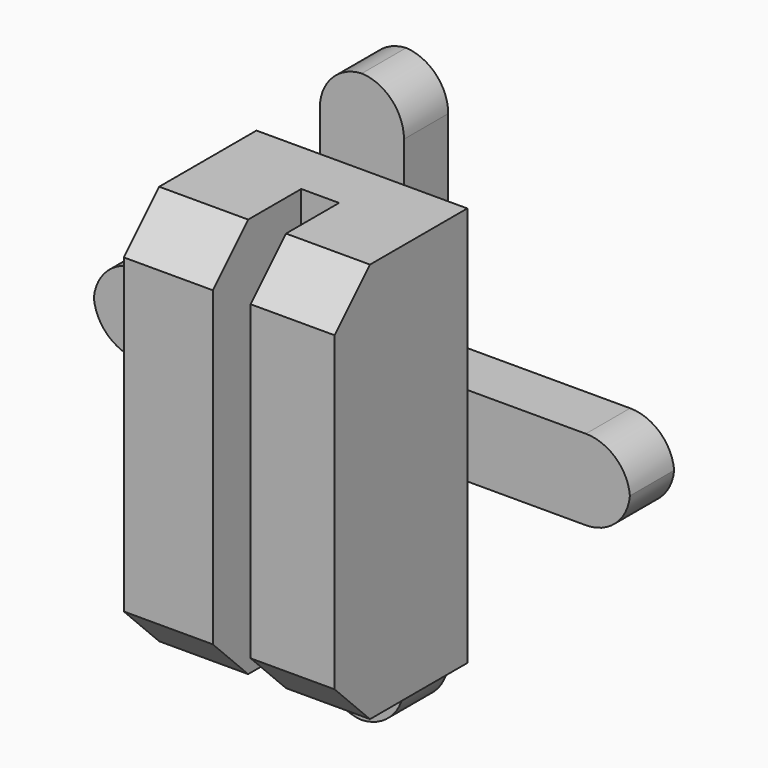
from build123d import *

# Parameters (mm, degrees)
F0_W        = 19.3394050002
F0_H        = 56.1432316899
F0_W_2      = 51.9402250648
F0_H_2      = 18.5019075871
F1_DEPTH    = 12.7
F2_T1_DEPTH = 63.5
F3_W        = 48.4298244119
F3_H        = 91.9232070446
F4_DEPTH    = 12.7
F5_W        = 20.4465882853
F5_H        = 91.9232070446
F5_W_2      = 19.2932416685
F6_DEPTH    = 25.4
F7_SIZE     = 10.16


# Not quite as in the source:
# - a fillet or chamfer that OpenCascade refuses, or shapes differently, is made with other operations: its cross-section is extruded or revolved along the edge and cut away or added


with BuildPart() as f1:
    # F0 (on Front) → F1 (new body)
    with BuildSketch(Plane.XZ):
        with Locations((0, 37.3225696385)):
            Rectangle(F0_W, F0_H)
        with Locations((35.6398150325, 0)):
            Rectangle(F0_W_2, F0_H_2)
        Rectangle(F0_W, F0_H_2)
        with Locations((-35.6398150325, 0)):
            Rectangle(F0_W_2, F0_H_2)
        with Locations((0, -37.3225696385)):
            Rectangle(F0_W, F0_H)
    extrude(amount=F1_DEPTH)

    # F2: fillet of radius 10.16 on 8 edges, made by hand

    # F2_s2 → F2_t1 (cut)
    with BuildSketch(Plane.XZ.offset(-25.4)):
        with BuildLine():
            ThreePointArc((9.6697025001, 55.2341854835), (6.693907397, 62.4183903803), (-0.4902974999, 65.3941854835))
            Line((-0.4902974999, 65.3941854835), (9.6697025001, 65.3941854835))
            Line((9.6697025001, 65.3941854835), (9.6697025001, 55.2341854835))
        make_face()
        with BuildLine():
            ThreePointArc((0.4902974999, 65.3941854835), (-6.693907397, 62.4183903803), (-9.6697025001, 55.2341854835))
            Line((-9.6697025001, 55.2341854835), (-9.6697025001, 65.3941854835))
            Line((-9.6697025001, 65.3941854835), (0.4902974999, 65.3941854835))
        make_face()
        with BuildLine():
            ThreePointArc((61.6099275649, -0.9090462065), (58.6341324617, 6.2751586904), (51.4499275649, 9.2509537935))
            Line((51.4499275649, 9.2509537935), (61.6099275649, 9.2509537935))
            Line((61.6099275649, 9.2509537935), (61.6099275649, -0.9090462065))
        make_face()
        with BuildLine():
            ThreePointArc((51.4499275649, -9.2509537935), (58.6341324617, -6.2751586904), (61.6099275649, 0.9090462065))
            Line((61.6099275649, 0.9090462065), (61.6099275649, -9.2509537935))
            Line((61.6099275649, -9.2509537935), (51.4499275649, -9.2509537935))
        make_face()
        with BuildLine():
            ThreePointArc((-0.4902974999, -65.3941854835), (6.693907397, -62.4183903803), (9.6697025001, -55.2341854835))
            Line((9.6697025001, -55.2341854835), (9.6697025001, -65.3941854835))
            Line((9.6697025001, -65.3941854835), (-0.4902974999, -65.3941854835))
        make_face()
        with BuildLine():
            ThreePointArc((-51.4499275649, 9.2509537935), (-58.6341324617, 6.2751586904), (-61.6099275649, -0.9090462065))
            Line((-61.6099275649, -0.9090462065), (-61.6099275649, 9.2509537935))
            Line((-61.6099275649, 9.2509537935), (-51.4499275649, 9.2509537935))
        make_face()
        with BuildLine():
            ThreePointArc((-61.6099275649, 0.9090462065), (-58.6341324617, -6.2751586904), (-51.4499275649, -9.2509537935))
            Line((-51.4499275649, -9.2509537935), (-61.6099275649, -9.2509537935))
            Line((-61.6099275649, -9.2509537935), (-61.6099275649, 0.9090462065))
        make_face()
        with BuildLine():
            ThreePointArc((-9.6697025001, -55.2341854835), (-6.693907397, -62.4183903803), (0.4902974999, -65.3941854835))
            Line((0.4902974999, -65.3941854835), (-9.6697025001, -65.3941854835))
            Line((-9.6697025001, -65.3941854835), (-9.6697025001, -55.2341854835))
        make_face()
    extrude(amount=F2_T1_DEPTH, mode=Mode.SUBTRACT)

    # F3 (on face) → F4 (join)
    with BuildSketch(Plane.XZ.offset(12.7)):
        Rectangle(F3_W, F3_H)
    extrude(amount=F4_DEPTH)

    # F5 (on face) → F6 (join)
    with BuildSketch(Plane.XZ.offset(25.4)):
        with Locations((-13.9916180633, 0)):
            Rectangle(F5_W, F5_H)
        with Locations((14.5682913717, 0)):
            Rectangle(F5_W_2, F5_H)
    extrude(amount=F6_DEPTH)

    # F7
    f7_edges = [f1.edges().sort_by_distance(p)[0] for p in [
        (-13.991618, -50.8, 45.961604),
        (-13.991618, -50.8, -45.961604),
        (14.568291, -50.8, -45.961604),
        (14.568291, -50.8, 45.961604),
    ]]
    chamfer(f7_edges, length=F7_SIZE)


solid = f1.part
